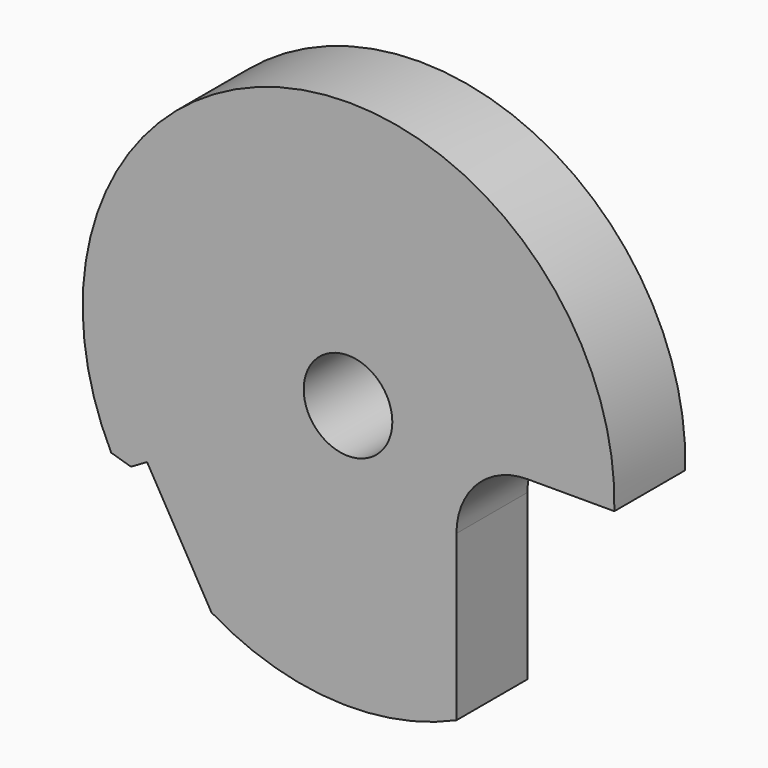
from build123d import *

# Parameters (mm, degrees)
F0_R        = 1.5875
F1_DEPTH    = 1.5875
F2_T1_DEPTH = 5.9319428422


# Not quite as in the source:
# - a fillet or chamfer that OpenCascade refuses, or shapes differently, is made with other operations: its cross-section is extruded or revolved along the edge and cut away or added


with BuildPart() as f1:
    # F0 (on Front) → F1 (new body, symmetric)
    with BuildSketch(Plane.XZ):
        with BuildLine():
            ThreePointArc((3.7381009291, -0.0336915449), (4.4820497049, 1.7623596793), (6.2781009291, 2.5063084551))
            Line((6.2781009291, 2.5063084551), (9.3939231872, 2.5063084551))
            ThreePointArc((9.3939231872, 2.5063084551), (-2.459861222, 12.0150971251), (-8.3760311943, -1.9823383417))
            Line((-8.3760311943, -1.9823383417), (-7.3443697718, -1.3867083417))
            Line((-7.3443697718, -1.3867083417), (-5.0381606197, -5.381179766))
            ThreePointArc((-5.0381606197, -5.381179766), (-0.7165786385, -6.7265825886), (3.7381009291, -5.9253276194))
            Line((3.7381009291, -5.9253276194), (3.7381009291, -0.0336915449))
        make_face()
        with Locations((-0.1472348195, 2.7336615811)):
            Circle(F0_R, mode=Mode.SUBTRACT)
    extrude(amount=F1_DEPTH, both=True)

    # F2: chamfer of 0.508 on 1 edges, made by hand

    # F2_s2 → F2_t1 (cut)
    with BuildSketch(Plane.XZ.offset(-2.9659714211)):
        with BuildLine():
            Line((-7.9236877385, -1.7211777257), (-8.6312397675, -1.5100480025))
            ThreePointArc((-8.6312397675, -1.5100480025), (-8.5103751964, -1.7416719985), (-8.3760311943, -1.9823383417))
            Line((-8.3760311943, -1.9823383417), (-7.9236877385, -1.7211777257))
        make_face()
    extrude(amount=F2_T1_DEPTH, mode=Mode.SUBTRACT)


solid = f1.part
